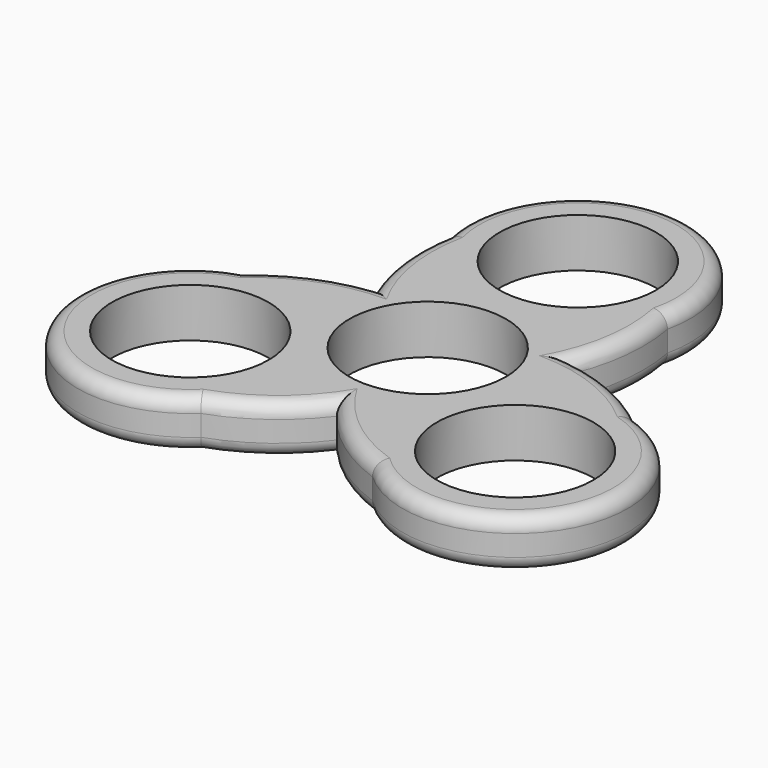
from build123d import *

# Parameters (mm, degrees)
F0_R     = 11.2
F1_DEPTH = 7
F3_R     = 2


# Not quite as in the source:
# - a feature of the source that left no trace in its solid (it failed there, or was rolled back) is left out


with BuildPart() as f1:
    # F0 (on Top) → F1 (new body)
    with BuildSketch(Plane.XY):
        with BuildLine():
            ThreePointArc((0, -16.2515131131), (5.4772663535, -21.648653647), (12.2815701726, -25.2306952695))
            ThreePointArc((12.2815701726, -25.2306952695), (37.2016797512, -21.4783998187), (27.9912081448, 1.9791958669))
            ThreePointArc((27.9912081448, 1.9791958669), (21.4869171927, 6.0808750181), (14.0742232059, 8.1257565566))
            ThreePointArc((14.0742232059, 8.1257565566), (16.0096508393, 15.5677786289), (15.7096379722, 23.2514994026))
            ThreePointArc((15.7096379722, 23.2514994026), (0, 42.9567996373), (-15.7096379722, 23.2514994026))
            ThreePointArc((-15.7096379722, 23.2514994026), (-16.0096508393, 15.5677786289), (-14.0742232059, 8.1257565566))
            ThreePointArc((-14.0742232059, 8.1257565566), (-21.4869171927, 6.0808750181), (-27.9912081448, 1.9791958669))
            ThreePointArc((-27.9912081448, 1.9791958669), (-37.2016797512, -21.4783998187), (-12.2815701726, -25.2306952695))
            ThreePointArc((-12.2815701726, -25.2306952695), (-5.4772663535, -21.648653647), (0, -16.2515131131))
        make_face()
        with Locations((-23.2459054754, -13.4210297838)):
            Circle(F0_R, mode=Mode.SUBTRACT)
        with Locations((23.2459054754, -13.4210297838)):
            Circle(F0_R, mode=Mode.SUBTRACT)
        Circle(F0_R, mode=Mode.SUBTRACT)
        with Locations((0, 26.8420595676)):
            Circle(F0_R, mode=Mode.SUBTRACT)
    extrude(amount=F1_DEPTH)

    # F3
    f3_edges = [f1.edges().sort_by_distance(p)[0] for p in [
        (0, 42.9568, 0),
        (21.486917, 6.080875, 0),
        (-37.20168, -21.4784, 0),
        (21.486917, 6.080875, 7),
        (0, 42.9568, 7),
        (-16.009651, 15.567779, 7),
        (-21.486917, 6.080875, 7),
        (-37.20168, -21.4784, 7),
        (-5.477266, -21.648654, 0),
        (-5.477266, -21.648654, 7),
        (5.477266, -21.648654, 0),
        (5.477266, -21.648654, 7),
        (37.20168, -21.4784, 0),
        (37.20168, -21.4784, 7),
        (16.009651, 15.567779, 0),
        (16.009651, 15.567779, 7),
        (-16.009651, 15.567779, 0),
        (-21.486917, 6.080875, 0),
    ]]
    fillet(f3_edges, radius=F3_R)


solid = f1.part
